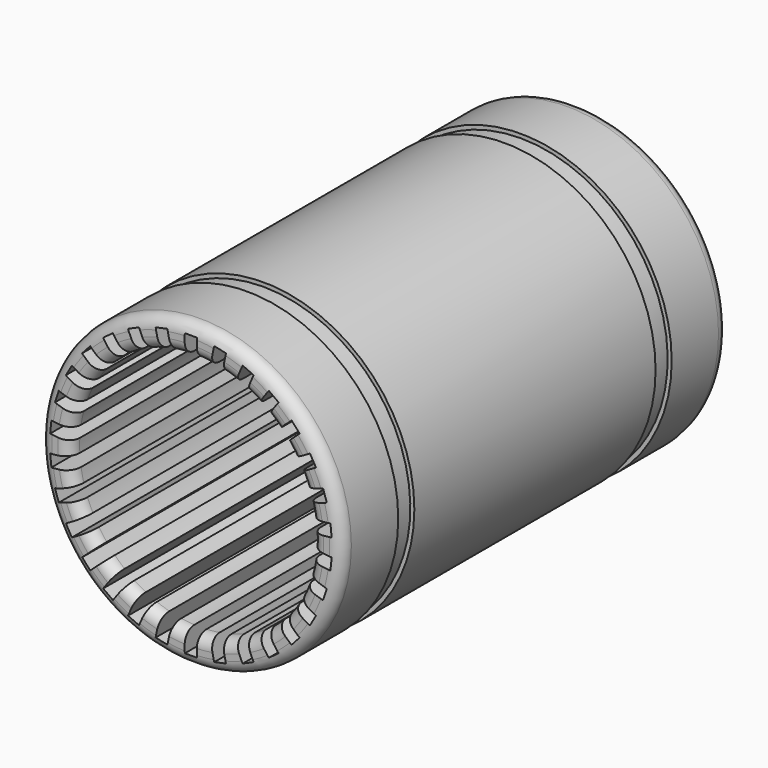
from build123d import *

# Parameters (mm, degrees)
F0_R          = 7.5
F0_R_2        = 6
F1_DEPTH      = 12
F2_R          = 0.6
F4_DEPTH      = 12.001
F4_DEPTH_BACK = 12.001
F6_COUNT      = 30
F7_W          = 1
F7_H          = 0.2


# Not quite as in the source:
# - a pattern or mirror of a feature is missing from the dataset's text; its kind, count and spacing are read off the source's solid


with BuildPart() as f1:
    # F0 (on Front) → F1 (new body, symmetric)
    with BuildSketch(Plane.XZ):
        Circle(F0_R)
        Circle(F0_R_2, mode=Mode.SUBTRACT)
    extrude(amount=F1_DEPTH, both=True)

    # F2
    f2_edges = [f1.edges().sort_by_distance(p)[0] for p in [
        (-6, -12, 0),
        (-7.5, -12, 0),
        (-6, 12, 0),
        (-7.5, 12, 0),
    ]]
    fillet(f2_edges, radius=F2_R)

    # F3 (on Front) → F4 (cut, two sides)
    with BuildSketch(Plane.XZ) as f4_sk:
        Polygon((-0.3, 0), (0, 0), (0.3, 0), (0.3, 7), (-0.3, 7), align=None)
    f4 = extrude(amount=-F4_DEPTH, mode=Mode.SUBTRACT) + extrude(f4_sk.sketch, amount=F4_DEPTH_BACK, mode=Mode.SUBTRACT)

    # F6: F4 ×30 about axis
    f6_axis = Axis((0, 0, 0), (0, 1, 0))
    for i in range(1, F6_COUNT):
        add(f4.rotate(f6_axis, i * 360 / F6_COUNT), mode=Mode.SUBTRACT)

    # F7 (on Right) → F8 (revolve, cut)
    with BuildSketch(Plane.YZ):
        with Locations((-7.9904858905, 7.4)):
            Rectangle(F7_W, F7_H)
    f8 = revolve(axis=Axis((0, 0.1834239811, 0), (0, 1, 0)), mode=Mode.SUBTRACT)

    # F8_copies: F8 across plane
    add(f8.mirror(Plane.ZX), mode=Mode.SUBTRACT)


solid = f1.part
